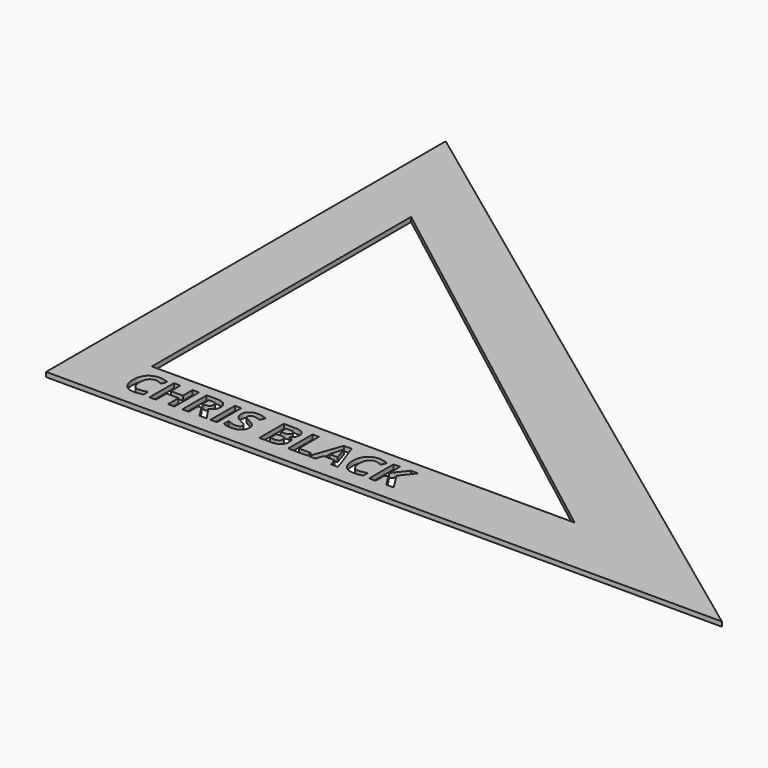
from build123d import *

# Parameters (mm, degrees)
F1_DEPTH     = 2
F2_SCALE     = 0.75
F3_TEXT_SIZE = 13.8751121122
F4_DEPTH     = 1.501


# Not quite as in the source:
# - Text() gives the source's letters only with a copy of the font that has no kerning and outlines rounded to 1/6400 em; it was checked with that copy


with BuildPart() as f1:
    # F0 (on Top) → F1 (new body)
    with BuildSketch(Plane.XY):
        Polygon((-110.3935540405, 109.5033976257), (-110.3935540405, -106.3966023743), (181.7064459595, -106.3966023743), align=None)
        Polygon((-84.9935540405, -80.9966023743), (-84.9935540405, 59.0477188125), (97.7188157638, -80.9966023743), align=None, mode=Mode.SUBTRACT)
    extrude(amount=F1_DEPTH)


with BuildPart() as f1_1:
    # F2: moved
    add(f1.part.scale(F2_SCALE))

    # F3 (on face) → F4 (cut, through all)
    with BuildSketch(Plane.XY.offset(1.5)):
        with Locations((-63.7451655304, -74.3297189474)):
            Text('CHRIS BLACK', F3_TEXT_SIZE, font='Open Sans', font_style=FontStyle.BOLD, text_align=(TextAlign.LEFT, TextAlign.BOTTOM))
    extrude(amount=-F4_DEPTH, mode=Mode.SUBTRACT)


solid = f1_1.part
